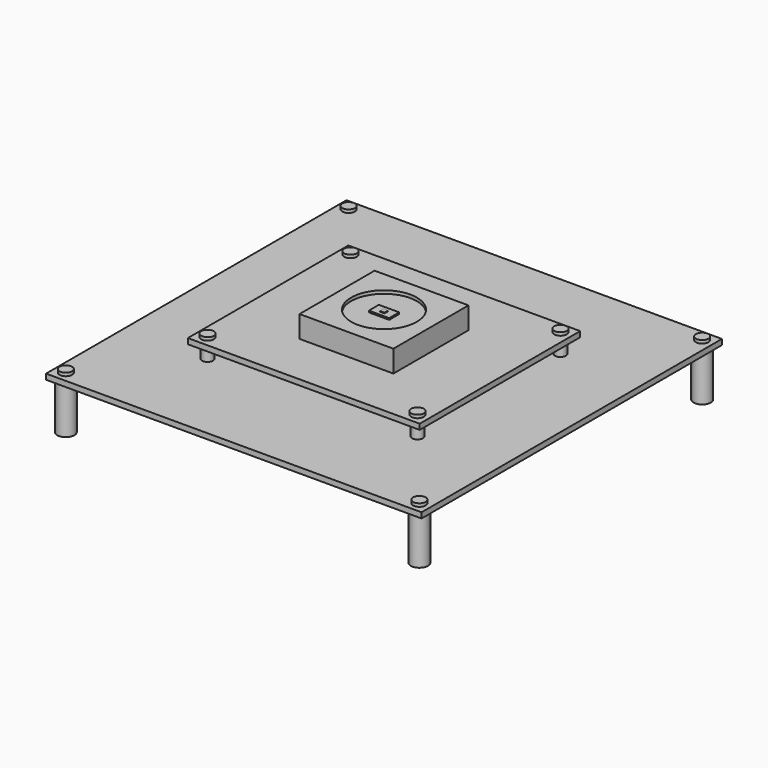
from build123d import *

# Parameters (mm, degrees)
F0_W      = 120
F0_H      = 120
F0_R      = 1.5
F1_DEPTH  = 1.75
F2_R      = 2.75
F2_R_2    = 1.5
F3_DEPTH  = 15
F4_R      = 2
F4_R_2    = 1.5
F5_DEPTH  = 1
F4_R_3    = 1.75
F6_DEPTH  = 4.35
F7_W      = 74.1
F7_H      = 64.1
F8_DEPTH  = 1.75
F9_R      = 2
F10_DEPTH = 1
F9_W      = 30
F9_H      = 30
F11_DEPTH = 7
F12_R     = 10.5
F12_W     = 6.5
F12_H     = 4
F13_DEPTH = 1
F12_W_2   = 1.5
F12_H_2   = 1.5
F14_DEPTH = 0.3
F15_DEPTH = 0.5


with BuildPart() as f1:
    # F0 (on Top) → F1 (new body)
    with BuildSketch(Plane.XY):
        Rectangle(F0_W, F0_H)
        with Locations((-56.5, -56.5)):
            Circle(F0_R, mode=Mode.SUBTRACT)
        with Locations((56.5, -56.5)):
            Circle(F0_R, mode=Mode.SUBTRACT)
        with Locations((-56.5, 56.5)):
            Circle(F0_R, mode=Mode.SUBTRACT)
        with Locations((56.5, 56.5)):
            Circle(F0_R, mode=Mode.SUBTRACT)
    extrude(amount=F1_DEPTH)

    # F2 (on face) → F3 (join)
    with BuildSketch(Plane(origin=(0, 0, 0), x_dir=(1, 0, 0), z_dir=(0, 0, -1))):
        with Locations((56.5, -56.5)):
            Circle(F2_R)
        with Locations((56.5, -56.5)):
            Circle(F2_R_2, mode=Mode.SUBTRACT)
        with Locations((-56.5, -56.5)):
            Circle(F2_R)
        with Locations((-56.5, -56.5)):
            Circle(F2_R_2, mode=Mode.SUBTRACT)
        with Locations((-56.5, 56.5)):
            Circle(F2_R)
        with Locations((-56.5, 56.5)):
            Circle(F2_R_2, mode=Mode.SUBTRACT)
        with Locations((56.5, 56.5)):
            Circle(F2_R)
        with Locations((56.5, 56.5)):
            Circle(F2_R_2, mode=Mode.SUBTRACT)
        with Locations((-56.5, 56.5)):
            Circle(F2_R_2)
        with Locations((56.5, 56.5)):
            Circle(F2_R_2)
        with Locations((-56.5, -56.5)):
            Circle(F2_R_2)
        with Locations((56.5, -56.5)):
            Circle(F2_R_2)
    extrude(amount=F3_DEPTH)

    # F4 (on face) → F5 (join)
    with BuildSketch(Plane.XY.offset(1.75)):
        with Locations((-56.5, 56.5)):
            Circle(F4_R)
        with Locations((-56.5, 56.5)):
            Circle(F4_R_2, mode=Mode.SUBTRACT)
        with Locations((-56.5, 56.5)):
            Circle(F4_R_2)
        with Locations((56.5, 56.5)):
            Circle(F4_R)
        with Locations((56.5, 56.5)):
            Circle(F4_R_2, mode=Mode.SUBTRACT)
        with Locations((56.5, 56.5)):
            Circle(F4_R_2)
        with Locations((56.5, -56.5)):
            Circle(F4_R)
        with Locations((56.5, -56.5)):
            Circle(F4_R_2, mode=Mode.SUBTRACT)
        with Locations((56.5, -56.5)):
            Circle(F4_R_2)
        with Locations((-56.5, -56.5)):
            Circle(F4_R)
        with Locations((-56.5, -56.5)):
            Circle(F4_R_2, mode=Mode.SUBTRACT)
        with Locations((-56.5, -56.5)):
            Circle(F4_R_2)
    extrude(amount=F5_DEPTH)

    # F4 (on face) → F6 (join)
    with BuildSketch(Plane.XY.offset(1.75)):
        with Locations((-33.55, -28.55)):
            Circle(F4_R_3)
        with Locations((33.55, -28.55)):
            Circle(F4_R_3)
        with Locations((33.55, 28.55)):
            Circle(F4_R_3)
        with Locations((-33.55, 28.55)):
            Circle(F4_R_3)
    extrude(amount=F6_DEPTH)

    # F7 (on face) → F8 (join)
    with BuildSketch(Plane.XY.offset(6.1)):
        Rectangle(F7_W, F7_H)
    extrude(amount=F8_DEPTH)

    # F9 (on face) → F10 (join)
    with BuildSketch(Plane.XY.offset(7.85)):
        with Locations((33.55, 28.55)):
            Circle(F9_R)
        with Locations((-33.55, 28.55)):
            Circle(F9_R)
        with Locations((33.55, -28.55)):
            Circle(F9_R)
        with Locations((-33.55, -28.55)):
            Circle(F9_R)
    extrude(amount=F10_DEPTH)

    # F9 (on face) → F11 (join)
    with BuildSketch(Plane.XY.offset(7.85)):
        Rectangle(F9_W, F9_H)
    extrude(amount=F11_DEPTH)

    # F12 (on face) → F13 (cut)
    with BuildSketch(Plane.XY.offset(14.85)):
        Circle(F12_R)
        Rectangle(F12_W, F12_H, mode=Mode.SUBTRACT)
    extrude(amount=-F13_DEPTH, mode=Mode.SUBTRACT)

    # F12 (on face) → F14 (cut)
    with BuildSketch(Plane.XY.offset(14.85)):
        Rectangle(F12_W_2, F12_H_2)
    extrude(amount=-F14_DEPTH, mode=Mode.SUBTRACT)

    # F12 (on face) → F15 (cut)
    with BuildSketch(Plane.XY.offset(14.85)):
        Rectangle(F12_W, F12_H)
        Rectangle(F12_W_2, F12_H_2, mode=Mode.SUBTRACT)
    extrude(amount=-F15_DEPTH, mode=Mode.SUBTRACT)


solid = f1.part
